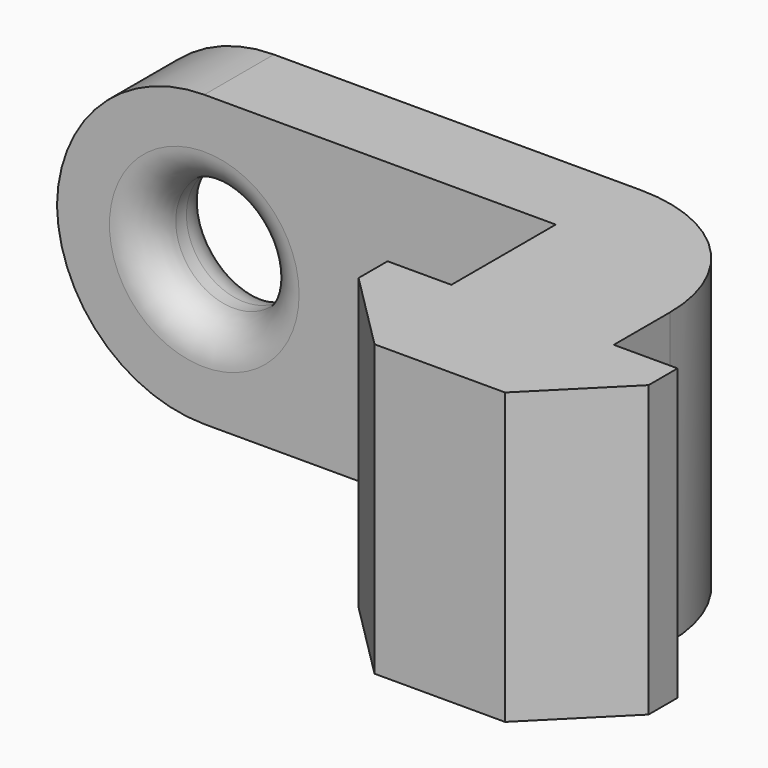
from build123d import *

# Parameters (mm, degrees)
F1_DEPTH    = 10
F2_R        = 5.08
F3_T1_DEPTH = 28.4
F4_R        = 2
F5_DEPTH    = 25.4
F6_R        = 1.27


# Not quite as in the source:
# - a fillet or chamfer that OpenCascade refuses, or shapes differently, is made with other operations: its cross-section is extruded or revolved along the edge and cut away or added


with BuildPart() as f1:
    # F0 (on Top) → F1 (new body)
    with BuildSketch(Plane.XY):
        Polygon((-2.25, -4), (0, -4), (2.25, -4), (5, -1.25), (5, 0), (2.8, 0), (2.8, 4), (2.8, 7.5), (-20, 7.5), (-20, 4.5), (-2.8, 4.5), (-2.8, 4), (-2.8, 0), (-5, 0), (-5, -1.25), align=None)
    extrude(amount=F1_DEPTH)

    # F2
    f2_edges = [f1.edges().sort_by_distance(p)[0] for p in [
        (2.8, 7.5, 5),
    ]]
    fillet(f2_edges, radius=F2_R)

    # F3: fillet of radius 5.08 on 2 edges, made by hand

    # F3_s2 → F3_t1 (cut)
    with BuildSketch(Plane.XZ.offset(-20.2)):
        with BuildLine():
            ThreePointArc((-20, 4.92), (-18.5121024484, 8.5121024484), (-14.92, 10))
            Line((-14.92, 10), (-20, 10))
            Line((-20, 10), (-20, 4.92))
        make_face()
        with BuildLine():
            ThreePointArc((-14.92, 0), (-18.5121024484, 1.4878975516), (-20, 5.08))
            Line((-20, 5.08), (-20, 0))
            Line((-20, 0), (-14.92, 0))
        make_face()
    extrude(amount=F3_T1_DEPTH, mode=Mode.SUBTRACT)

    # F4 (on face) → F5 (cut)
    with BuildSketch(Plane.XZ.offset(-4.5)):
        with Locations((-14.92, 5)):
            Circle(F4_R)
    extrude(amount=-F5_DEPTH, mode=Mode.SUBTRACT)

    # F6
    f6_edges = [f1.edges().sort_by_distance(p)[0] for p in [
        (-16.92, 4.5, 5),
        (-16.92, 7.5, 5),
    ]]
    fillet(f6_edges, radius=F6_R)


solid = f1.part
